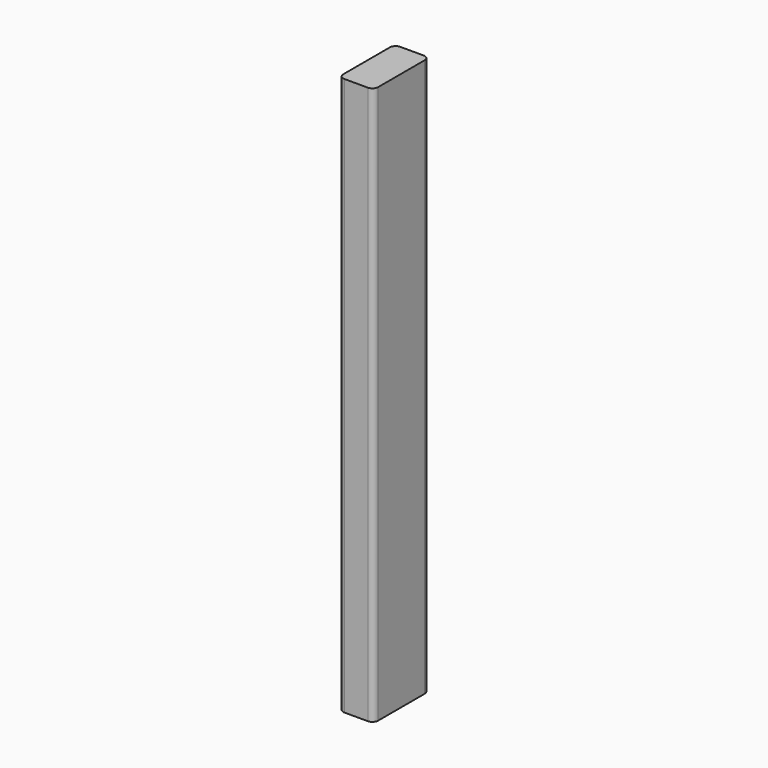
from build123d import *

# Parameters (mm, degrees)
F1_DEPTH = 304.8


# Not quite as in the source:
# - a feature names something its author has since deleted; it is built from what else it names


with BuildPart() as f1:
    # F0 (on Top) → F1 (new body)
    with BuildSketch(Plane.XY):
        with BuildLine():
            Line((19.05, 34.9504), (19.05, 3.1496))
            ThreePointArc((19.05, 3.1496), (19.972496482, 0.922496482), (22.1996, 0))
            Line((22.1996, 0), (34.9504, 0))
            ThreePointArc((34.9504, 0), (37.177503518, 0.922496482), (38.1, 3.1496))
            Line((38.1, 3.1496), (38.1, 34.9504))
            ThreePointArc((38.1, 34.9504), (37.177503518, 37.177503518), (34.9504, 38.1))
            Line((34.9504, 38.1), (22.1996, 38.1))
            ThreePointArc((22.1996, 38.1), (19.972496482, 37.177503518), (19.05, 34.9504))
        make_face()
    extrude(amount=F1_DEPTH)


solid = f1.part
